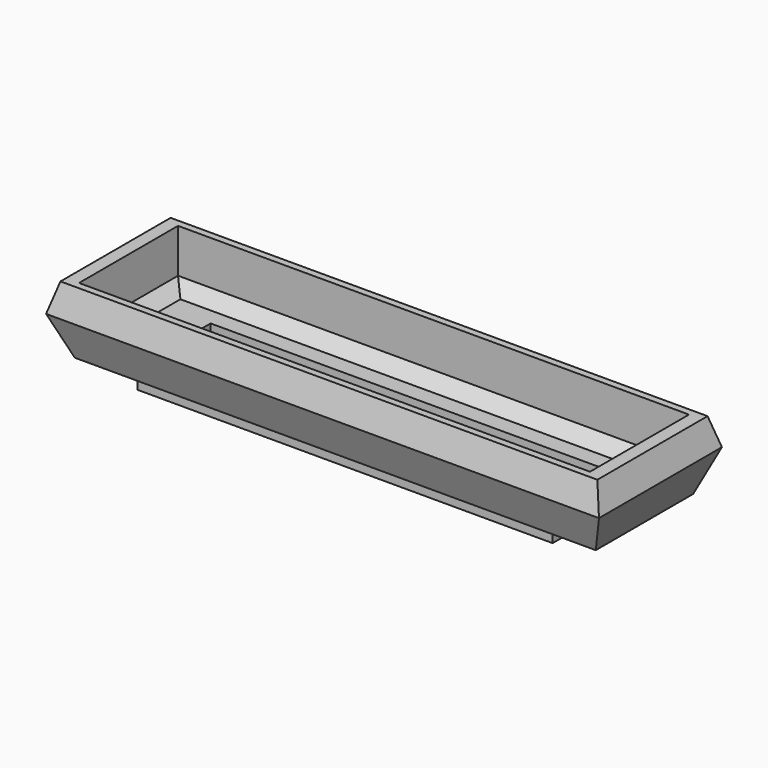
from build123d import *

# Parameters (mm, degrees)
F0_W      = 69.25
F0_H      = 19.25
F1_DEPTH  = 8.5
F3_SIZE2  = 1
F3_SIZE   = 3.5
F4_SIZE2  = 4.99999
F4_SIZE   = 1.99999
F2_W      = 64
F2_H      = 15.5
F5_DEPTH  = 7
F6_W      = 52
F6_H      = 12.2
F7_DEPTH  = 2
F8_W      = 7.9
F8_H      = 7.7
F8_H_2    = 2.2
F9_DEPTH  = 2
F8_W_2    = 13.4
F8_H_3    = 5.4
F10_DEPTH = 25
F11_W     = 50
F11_H     = 8.2
F11_W_2   = 13.4
F11_H_2   = 5.4
F11_H_3   = 5.3
F12_DEPTH = 1.5
F13_SIZE  = 1.5


# Not quite as in the source:
# - a fillet or chamfer is up to 0.001 mm smaller than in the source, because OpenCascade refuses the exact size


with BuildPart() as f1:
    # F0 (on Top) → F1 (new body)
    with BuildSketch(Plane.XY):
        Rectangle(F0_W, F0_H)
    extrude(amount=F1_DEPTH)

    # F3
    f3_edges = [f1.edges().sort_by_distance(p)[0] for p in [
        (-34.625, 0, 8.5),
        (0, -9.625, 8.5),
        (34.625, 0, 8.5),
        (0, 9.625, 8.5),
    ]]
    chamfer(f3_edges, length=F3_SIZE, length2=F3_SIZE2)

    # F4 (size 2 and 5 in the source; OpenCascade refuses exactly that, so slightly less here)
    f4_edges = [f1.edges().sort_by_distance(p)[0] for p in [
        (-34.625, 0, 0),
        (0, -9.625, 0),
        (0, 9.625, 0),
        (34.625, 0, 0),
    ]]
    f4_side = f1.faces().sort_by_distance((0, 0, 0))[0]
    chamfer(f4_edges, length=F4_SIZE, length2=F4_SIZE2, reference=f4_side)

    # F2 (on face) → F5 (cut)
    with BuildSketch(Plane.XY.offset(8.5)):
        Rectangle(F2_W, F2_H)
    extrude(amount=-F5_DEPTH, mode=Mode.SUBTRACT)

    # F6 (on face) → F7 (join)
    with BuildSketch(Plane(origin=(0, 0, 0), x_dir=(1, 0, 0), z_dir=(0, 0, -1))):
        Rectangle(F6_W, F6_H)
    extrude(amount=F7_DEPTH)

    # F8 (on face) → F9 (cut)
    with BuildSketch(Plane(origin=(0, 0, -2), x_dir=(1, 0, 0), z_dir=(0, 0, -1))):
        with Locations((0, -1.1)):
            Rectangle(F8_W, F8_H)
        with Locations((0, 3.85)):
            Rectangle(F8_W, F8_H_2)
    extrude(amount=-F9_DEPTH, mode=Mode.SUBTRACT)

    # F8 (on face) → F10 (cut)
    with BuildSketch(Plane(origin=(0, 0, -2), x_dir=(1, 0, 0), z_dir=(0, 0, -1))):
        with Locations((-15.9, 0.05)):
            Rectangle(F8_W_2, F8_H_3)
        Polygon((15.7195143402, 2.75), (9.2, 2.75), (9.2, -2.55), (22.6, -2.55), (22.6, 2.75), align=None)
    extrude(amount=-F10_DEPTH, mode=Mode.SUBTRACT)

    # F11 (on face) → F12 (cut)
    with BuildSketch(Plane.XY.offset(1.5)):
        Rectangle(F11_W, F11_H)
        with Locations((-15.9, -0.05)):
            Rectangle(F11_W_2, F11_H_2, mode=Mode.SUBTRACT)
        with Locations((15.9, -0.1)):
            Rectangle(F11_W_2, F11_H_3, mode=Mode.SUBTRACT)
    extrude(amount=-F12_DEPTH, mode=Mode.SUBTRACT)

    # F13
    f13_edges = [f1.edges().sort_by_distance(p)[0] for p in [
        (-32, 0, 1.5),
        (0, 7.75, 1.5),
        (32, 0, 1.5),
        (0, -7.75, 1.5),
    ]]
    chamfer(f13_edges, length=F13_SIZE)


solid = f1.part
